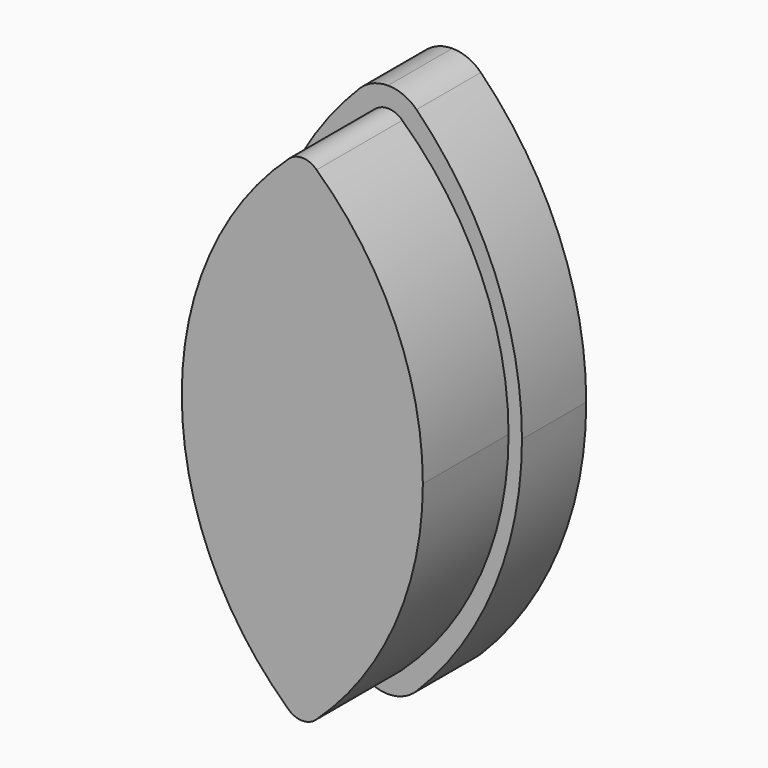
from build123d import *

# Parameters (mm, degrees)
F1_DEPTH = 6
F3_DEPTH = 8


with BuildPart() as f1:
    # F0 (on Front) → F1 (new body)
    with BuildSketch(Plane.XZ):
        with BuildLine():
            ThreePointArc((7.8698224852, 39.1124260355), (2.0444516128, 30.3346375712), (0, 20))
            Line((0, 20), (10, 20))
            Line((10, 20), (10, 34))
            ThreePointArc((10, 34), (7.2307692308, 35.8461538462), (7.8698224852, 39.1124260355))
        make_face()
        with BuildLine():
            Line((10, 34), (10, 20))
            Line((10, 20), (20, 20))
            ThreePointArc((20, 20), (17.9555483872, 30.3346375712), (12.1301775148, 39.1124260355))
            ThreePointArc((12.1301775148, 39.1124260355), (12.7740342954, 38.1422494158), (13, 37))
            ThreePointArc((13, 37), (12.1213203436, 34.8786796564), (10, 34))
        make_face()
        with BuildLine():
            Line((10, 20), (0, 20))
            ThreePointArc((0, 20), (2.0444516128, 9.6653624288), (7.8698224852, 0.8875739645))
            ThreePointArc((7.8698224852, 0.8875739645), (7.2307692308, 4.1538461538), (10, 6))
            Line((10, 6), (10, 20))
        make_face()
        with BuildLine():
            Line((10, 20), (10, 6))
            ThreePointArc((10, 6), (12.1213203436, 5.1213203436), (13, 3))
            ThreePointArc((13, 3), (12.7740342954, 1.8577505842), (12.1301775148, 0.8875739645))
            ThreePointArc((12.1301775148, 0.8875739645), (17.9555483872, 9.6653624288), (20, 20))
            Line((20, 20), (10, 20))
        make_face()
        with BuildLine():
            ThreePointArc((7.8698224852, 0.8875739645), (8.8461538462, 0.2307692308), (10, 0))
            Line((10, 0), (10, 6))
            ThreePointArc((10, 6), (7.2307692308, 4.1538461538), (7.8698224852, 0.8875739645))
        make_face()
        with BuildLine():
            Line((10, 6), (10, 0))
            ThreePointArc((10, 0), (11.1538461538, 0.2307692308), (12.1301775148, 0.8875739645))
            ThreePointArc((12.1301775148, 0.8875739645), (12.7740342954, 1.8577505842), (13, 3))
            ThreePointArc((13, 3), (12.1213203436, 5.1213203436), (10, 6))
        make_face()
        with BuildLine():
            ThreePointArc((10, 40), (8.8461538462, 39.7692307692), (7.8698224852, 39.1124260355))
            ThreePointArc((7.8698224852, 39.1124260355), (7.2307692308, 35.8461538462), (10, 34))
            Line((10, 34), (10, 40))
        make_face()
        with BuildLine():
            ThreePointArc((12.1301775148, 39.1124260355), (11.1538461538, 39.7692307692), (10, 40))
            Line((10, 40), (10, 34))
            ThreePointArc((10, 34), (12.1213203436, 34.8786796564), (13, 37))
            ThreePointArc((13, 37), (12.7740342954, 38.1422494158), (12.1301775148, 39.1124260355))
        make_face()
    extrude(amount=F1_DEPTH)

    # F2 (on face) → F3 (join)
    with BuildSketch(Plane.XZ.offset(6)):
        with BuildLine():
            ThreePointArc((8.9349112426, 1.9437869822), (10, 1.5), (11.0650887574, 1.9437869822))
            ThreePointArc((11.0650887574, 1.9437869822), (16.5685312395, 10.2364871367), (18.5, 20))
            Line((18.5, 20), (2.4724225514, 20))
            Line((2.4724225514, 20), (1.5, 20))
            ThreePointArc((1.5, 20), (3.4314687605, 10.2364871367), (8.9349112426, 1.9437869822))
        make_face()
        with BuildLine():
            Line((2.4724225514, 20), (18.5, 20))
            ThreePointArc((18.5, 20), (16.5685312395, 29.7635128633), (11.0650887574, 38.0562130178))
            ThreePointArc((11.0650887574, 38.0562130178), (10, 38.5), (8.9349112426, 38.0562130178))
            ThreePointArc((8.9349112426, 38.0562130178), (3.4314687605, 29.7635128633), (1.5, 20))
            Line((1.5, 20), (2.4724225514, 20))
        make_face()
        with BuildLine():
            ThreePointArc((18.5, 20), (16.5685312395, 10.2364871367), (11.0650887574, 1.9437869822))
            ThreePointArc((11.0650887574, 1.9437869822), (16.9287608071, 10.1385897944), (19, 20))
            Line((19, 20), (18.5, 20))
        make_face()
        with BuildLine():
            ThreePointArc((11.0650887574, 38.0562130178), (16.5685312395, 29.7635128633), (18.5, 20))
            Line((18.5, 20), (19, 20))
            ThreePointArc((19, 20), (16.9287608071, 29.8614102056), (11.0650887574, 38.0562130178))
        make_face()
        with BuildLine():
            ThreePointArc((1, 20), (3.0712391929, 10.1385897944), (8.9349112426, 1.9437869822))
            ThreePointArc((8.9349112426, 1.9437869822), (3.4314687605, 10.2364871367), (1.5, 20))
            Line((1.5, 20), (1, 20))
        make_face()
        with BuildLine():
            Line((1, 20), (1.5, 20))
            ThreePointArc((1.5, 20), (3.4314687605, 29.7635128633), (8.9349112426, 38.0562130178))
            ThreePointArc((8.9349112426, 38.0562130178), (3.0712391929, 29.8614102056), (1, 20))
        make_face()
    extrude(amount=F3_DEPTH)


solid = f1.part
